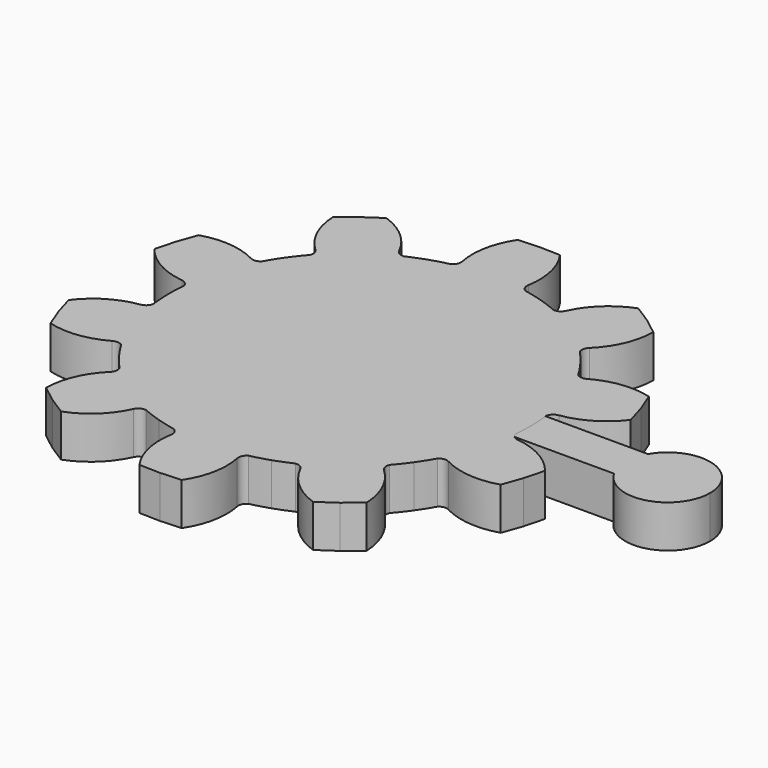
from build123d import *

# Parameters (mm, degrees)
F4_DEPTH = 10
F7_DEPTH = 10
F8_COUNT = 10


# Not quite as in the source:
# - a feature names something its author has since deleted; it is built from what else it names


with BuildPart() as f4:
    # F3 (on Top) → F4 (new body)
    with BuildSketch(Plane.XY):
        with BuildLine():
            Line((0, 5), (8.6602540378, 5))
            ThreePointArc((8.6602540378, 5), (-10, 0), (8.6602540378, -5))
            Line((8.6602540378, -5), (0, -5))
            Line((0, -5), (0, 5))
        make_face()
        with BuildLine():
            ThreePointArc((8.6602540378, 5), (9.6592582629, 2.588190451), (10, 0))
            ThreePointArc((10, 0), (9.6592582629, -2.588190451), (8.6602540378, -5))
            Line((8.6602540378, -5), (66.3397459622, -5))
            ThreePointArc((66.3397459622, -5), (65, 0), (66.3397459622, 5))
            Line((66.3397459622, 5), (8.6602540378, 5))
        make_face()
        with BuildLine():
            ThreePointArc((85, 0), (77.588190451, 9.6592582629), (66.3397459622, 5))
            Line((66.3397459622, 5), (75, 5))
            Line((75, 5), (75, -5))
            Line((75, -5), (66.3397459622, -5))
            ThreePointArc((66.3397459622, -5), (77.588190451, -9.6592582629), (85, 0))
        make_face()
        with BuildLine():
            Line((75, 5), (66.3397459622, 5))
            ThreePointArc((66.3397459622, 5), (65, 0), (66.3397459622, -5))
            Line((66.3397459622, -5), (75, -5))
            Line((75, -5), (75, 5))
        make_face()
        with BuildLine():
            ThreePointArc((8.6602540378, -5), (9.6592582629, -2.588190451), (10, 0))
            ThreePointArc((10, 0), (9.6592582629, 2.588190451), (8.6602540378, 5))
            Line((8.6602540378, 5), (0, 5))
            Line((0, 5), (0, -5))
            Line((0, -5), (8.6602540378, -5))
        make_face()
    extrude(amount=F4_DEPTH)


with BuildPart() as f7:
    # F5 (on Top) → F7 (new body)
    with BuildSketch(Plane.XY):
        with BuildLine():
            ThreePointArc((-13.7207679114, 40.2242529815), (-24.7297125313, -34.5643069961), (42.5, 0))
            ThreePointArc((42.5, 0), (34.2003125005, 25.2307079739), (12.5428882416, 40.6069692855))
            Line((12.5428882416, 40.6069692855), (8.5840838738, 41.526906744))
            ThreePointArc((8.5840838738, 41.526906744), (8.3163788428, 41.6092495204), (8.0628019611, 41.7281826172))
            ThreePointArc((8.0628019611, 41.7281826172), (-0.6192479887, 42.4954883715), (-9.2752537824, 41.4755309462))
            ThreePointArc((-9.2752537824, 41.4755309462), (-9.5252575239, 41.3492596284), (-9.7904495841, 41.2591514287))
            Line((-9.7904495841, 41.2591514287), (-13.7207679114, 40.2242529815))
        make_face()
        with BuildLine():
            Line((8.5840838738, 41.526906744), (12.5428882416, 40.6069692855))
            ThreePointArc((12.5428882416, 40.6069692855), (10.3180859183, 41.2284744198), (8.0628019611, 41.7281826172))
            ThreePointArc((8.0628019611, 41.7281826172), (8.3163788428, 41.6092495204), (8.5840838738, 41.526906744))
        make_face()
        with BuildLine():
            ThreePointArc((-9.2752537824, 41.4755309462), (-11.5150196514, 40.910320488), (-13.7207679114, 40.2242529815))
            Line((-13.7207679114, 40.2242529815), (-9.7904495841, 41.2591514287))
            ThreePointArc((-9.7904495841, 41.2591514287), (-9.5252575239, 41.3492596284), (-9.2752537824, 41.4755309462))
        make_face()
        with BuildLine():
            ThreePointArc((-9.2752537824, 41.4755309462), (-0.6192479887, 42.4954883715), (8.0628019611, 41.7281826172))
            ThreePointArc((8.0628019611, 41.7281826172), (7.2325873296, 42.6119250894), (7.0655284339, 43.8129031978))
            ThreePointArc((7.0655284339, 43.8129031978), (6.8828970608, 50.6273818317), (4.1037621109, 56.8520811979))
            Line((4.1037621109, 56.8520811979), (-0.8305208318, 56.99394911))
            Line((-0.8305208318, 56.99394911), (-5.758574926, 56.7083663565))
            ThreePointArc((-5.758574926, 56.7083663565), (-8.3551546341, 50.4053316041), (-8.3391482628, 43.5884248961))
            ThreePointArc((-8.3391482628, 43.5884248961), (-8.471142139, 42.3830889644), (-9.2752537824, 41.4755309462))
        make_face()
    extrude(amount=F7_DEPTH)

    # F8: F7 ×10 about axis
    f8_axis = Axis((0, 0, -2.4173539132), (0, 0, 1))


with BuildPart() as f7_1:
    add(f7.part)
    for i in range(1, F8_COUNT):
        add(f7.part.rotate(f8_axis, i * 360 / F8_COUNT))


solid = Compound([f4.part, f7_1.part])
